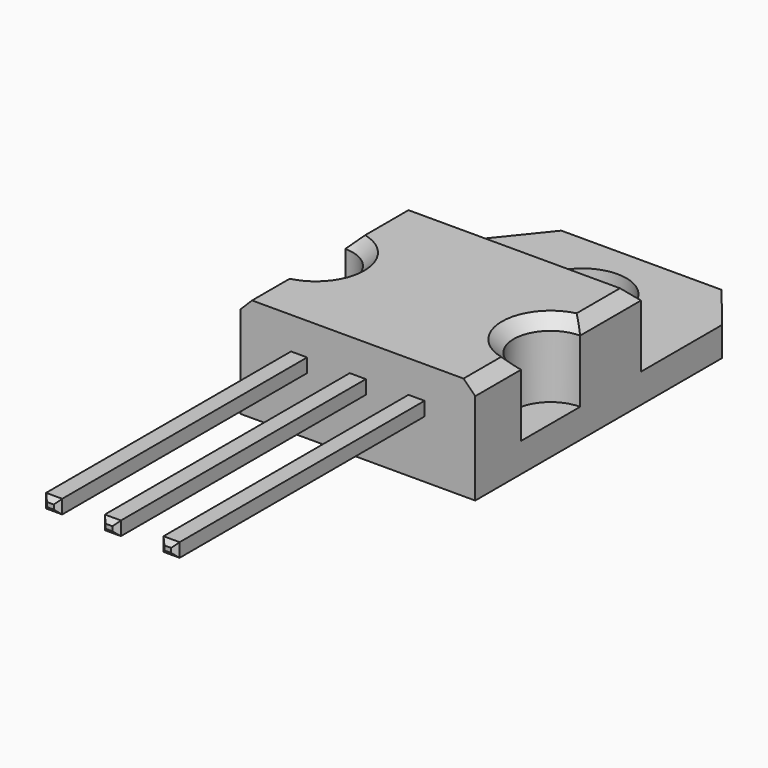
from build123d import *

# Parameters (mm, degrees)
F1_DEPTH = 4.5
F0_R     = 1.9
F2_DEPTH = 1.27
F3_SIZE  = 0.508
F4_W     = 0.7
F4_H     = 0.6
F5_DEPTH = 13.5
F6_SIZE  = 0.2032


with BuildPart() as f1:
    # F0 (on Top) → F1 (new body)
    with BuildSketch(Plane.XY):
        with BuildLine():
            Line((5.1, -2.006139996), (5.1, 1.3))
            Line((5.1, 1.3), (-5.1, 1.3))
            Line((-5.1, 1.3), (-5.1, -2.006139996))
            ThreePointArc((-5.1, -2.006139996), (-3.4965183315, -3.6096216645), (-5.1, -5.213103333))
            Line((-5.1, -5.213103333), (-5.1, -7.7))
            Line((-5.1, -7.7), (5.1, -7.7))
            Line((5.1, -7.7), (5.1, -5.213103333))
            ThreePointArc((5.1, -5.213103333), (3.4965183315, -3.6096216645), (5.1, -2.006139996))
        make_face()
    extrude(amount=F1_DEPTH)

    # F0 (on Top) → F2 (join)
    with BuildSketch(Plane.XY):
        Polygon((5.1, 5.6912479922), (3.4809927456, 7.7), (-3.4809927456, 7.7), (-5.1, 5.6912479922), (-5.1, 1.3), (5.1, 1.3), align=None)
        with Locations((0, 4.5)):
            Circle(F0_R, mode=Mode.SUBTRACT)
        with BuildLine():
            ThreePointArc((-5.1, -5.213103333), (-3.4965183315, -3.6096216645), (-5.1, -2.006139996))
            Line((-5.1, -2.006139996), (-5.1, -5.213103333))
        make_face()
        with BuildLine():
            Line((5.1, -5.213103333), (5.1, -2.006139996))
            ThreePointArc((5.1, -2.006139996), (3.4965183315, -3.6096216645), (5.1, -5.213103333))
        make_face()
    extrude(amount=F2_DEPTH)

    # F3
    f3_edges = [f1.edges().sort_by_distance(p)[0] for p in [
        (-5.1, -6.456552, 4.5),
        (0, 1.3, 4.5),
        (5.1, -0.35307, 4.5),
        (3.496518, -3.609622, 4.5),
        (-3.496518, -3.609622, 4.5),
        (5.1, -6.456552, 4.5),
        (-5.1, -0.35307, 4.5),
    ]]
    chamfer(f3_edges, length=F3_SIZE)

    # F4 (on face) → F5 (join)
    with BuildSketch(Plane.XZ.offset(7.7)):
        with Locations((-2.55, 2.8)):
            Rectangle(F4_W, F4_H)
        with Locations((0, 2.8)):
            Rectangle(F4_W, F4_H)
        with Locations((2.55, 2.8)):
            Rectangle(F4_W, F4_H)
    extrude(amount=F5_DEPTH)

    # F6
    f6_edges = [f1.edges().sort_by_distance(p)[0] for p in [
        (-2.55, -21.2, 3.1),
        (-2.9, -21.2, 2.8),
        (-2.55, -21.2, 2.5),
        (-2.2, -21.2, 2.8),
        (0, -21.2, 3.1),
        (-0.35, -21.2, 2.8),
        (0, -21.2, 2.5),
        (0.35, -21.2, 2.8),
        (2.55, -21.2, 3.1),
        (2.2, -21.2, 2.8),
        (2.55, -21.2, 2.5),
        (2.9, -21.2, 2.8),
    ]]
    chamfer(f6_edges, length=F6_SIZE)


solid = f1.part
